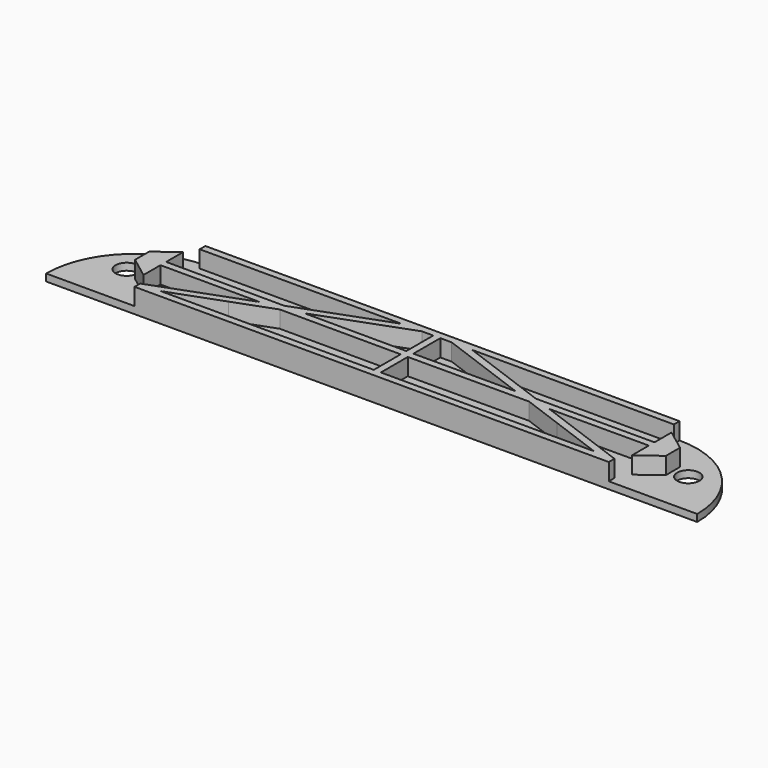
from build123d import *

# Parameters (mm, degrees)
F1_DEPTH = 6.8
F2_T     = -2
F4_DEPTH = 4.8
F6_DEPTH = 4.8
F5_R     = 3.15
F7_DEPTH = 2


# Not quite as in the source:
# - a feature names something its author has since deleted; it is built from what else it names


with BuildPart() as f1:
    # F0 (on Top) → F1 (new body)
    with BuildSketch(Plane.XY):
        with BuildLine():
            Line((129.8559711718, 33.7323809788), (-4.1440288282, 33.7323809788))
            ThreePointArc((-4.1440288282, 33.7323809788), (-21.8216983579, 26.4100505084), (-29.1440288282, 8.7323809788))
            Line((-29.1440288282, 8.7323809788), (154.8559711718, 8.7323809788))
            ThreePointArc((154.8559711718, 8.7323809788), (147.5336407015, 26.4100505084), (129.8559711718, 33.7323809788))
        make_face()
    extrude(amount=F1_DEPTH)

    # F2
    f2_openings = [f1.faces().sort_by_distance(p)[0] for p in [
        (62.855971, 20.804106, 6.8),
    ]]
    offset(amount=F2_T, openings=f2_openings)

    # F3 (on face) → F4 (cut)
    with BuildSketch(Plane.XY.offset(6.8)):
        with BuildLine():
            Line((-4.1440288282, 8.7323809788), (-4.1440288282, 10.7323809788))
            Line((-4.1440288282, 10.7323809788), (-27.056907303, 10.7323809788))
            ThreePointArc((-27.056907303, 10.7323809788), (-19.6842990961, 25.6882059366), (-4.1440288282, 31.7323809788))
            Line((-4.1440288282, 31.7323809788), (-4.1440288282, 33.7323809788))
            ThreePointArc((-4.1440288282, 33.7323809788), (-21.8216983579, 26.4100505084), (-29.1440288282, 8.7323809788))
            Line((-29.1440288282, 8.7323809788), (-4.1440288282, 8.7323809788))
        make_face()
        with BuildLine():
            Line((152.7688496466, 10.7323809788), (129.8559711718, 10.7323809788))
            Line((129.8559711718, 10.7323809788), (129.8559711718, 8.7323809788))
            Line((129.8559711718, 8.7323809788), (154.8559711718, 8.7323809788))
            ThreePointArc((154.8559711718, 8.7323809788), (147.5336407015, 26.4100505084), (129.8559711718, 33.7323809788))
            Line((129.8559711718, 33.7323809788), (129.8559711718, 31.7323809788))
            ThreePointArc((129.8559711718, 31.7323809788), (145.3962414397, 25.6882059366), (152.7688496466, 10.7323809788))
        make_face()
    extrude(amount=-F4_DEPTH, mode=Mode.SUBTRACT)

    # F5 (on face) → F6 (join)
    with BuildSketch(Plane.XY.offset(2)):
        Polygon((-6.1442747528, 21.3878121691), (-6.144358997, 22.3878121656), (-6.1448644621, 28.3878121443), (-12.1442590792, 23.9015265012), (-12.1442590792, 21.4015265012), (-12.1442590792, 18.9015265012), (-6.1442747528, 14.3878121691), (-6.1442747528, 20.3878121691), align=None)
        Polygon((21.8896443518, 20.3237342556), (27.2847434124, 22.3114023306), (-6.144358997, 22.3878121656), (-6.1442747528, 21.3878121691), (-6.1442747528, 20.3878121691), align=None)
        Polygon((-4.1440288282, 10.7323809788), (1.6412445236, 10.7323809788), (16.3966900356, 16.1685977463), (27.6392464887, 20.3105922291), (21.8896443518, 20.3237342556), align=None)
        Polygon((32.9729093256, 22.2756259058), (33.0343455494, 22.298260304), (27.2847434124, 22.3114023306), (21.8896443518, 20.3237342556), (27.6392464887, 20.3105922291), align=None)
        Polygon((33.0343455494, 22.298260304), (58.6412445236, 31.7323809788), (54.8559711718, 31.7323809788), (52.8559711718, 31.7323809788), (27.2847434124, 22.3114023306), align=None)
        Polygon((61.8564633663, 20.2323809788), (61.8564633663, 22.2323807827), (33.0343455494, 22.298260304), (32.9729093256, 22.2756259058), (27.6392464887, 20.3105922291), align=None)
        Polygon((62.8559711718, 10.7323809788), (62.8559711718, 31.7323809788), (61.8564633663, 31.7323809788), (61.8564633663, 22.2323807827), (61.8564633663, 20.2323809788), (61.8564633663, 10.7323809788), align=None)
        Polygon((92.6775967943, 22.298260304), (63.8559711718, 22.2323819077), (63.8559711718, 20.2323821038), (98.0726958549, 20.3105922291), (92.7390330181, 22.2756259058), align=None)
        Polygon((72.8559711718, 31.7323809788), (67.07069782, 31.7323809788), (92.6775967943, 22.298260304), (98.4271989312, 22.3114023306), align=None)
        Polygon((98.4271989312, 22.3114023306), (92.6775967943, 22.298260304), (92.7390330181, 22.2756259058), (98.0726958549, 20.3105922291), (103.8222979918, 20.3237342556), align=None)
        Polygon((109.3152523081, 16.1685977463), (124.07069782, 10.7323809788), (129.8559711718, 10.7323809788), (103.8222979918, 20.3237342556), (98.0726958549, 20.3105922291), align=None)
        Polygon((131.8563013406, 22.3878121656), (98.4271989312, 22.3114023306), (103.8222979918, 20.3237342556), (131.8562170965, 20.3878121691), (131.8562170965, 21.3878121691), align=None)
        Polygon((131.8568068057, 28.3878121443), (131.8563013406, 22.3878121656), (131.8562170965, 21.3878121691), (131.8562170965, 20.3878121691), (131.8562170965, 14.3878121691), (137.8562014229, 18.9015265012), (137.8562014229, 21.4015265012), (137.8562014229, 23.9015265012), align=None)
        Polygon((63.8559711718, 31.7323809788), (62.8559711718, 31.7323809788), (62.8559711718, 10.7323809788), (63.8559711718, 10.7323809788), (63.8559711718, 20.2323821038), (63.8559711718, 22.2323819077), align=None)
    extrude(amount=F6_DEPTH)

    # F5 (on face) → F7 (cut)
    with BuildSketch(Plane.XY.offset(2)):
        with Locations((-16.4942590792, 21.4015265012)):
            Circle(F5_R)
        with Locations((142.2062014229, 21.4015265012)):
            Circle(F5_R)
    extrude(amount=-F7_DEPTH, mode=Mode.SUBTRACT)


solid = f1.part
